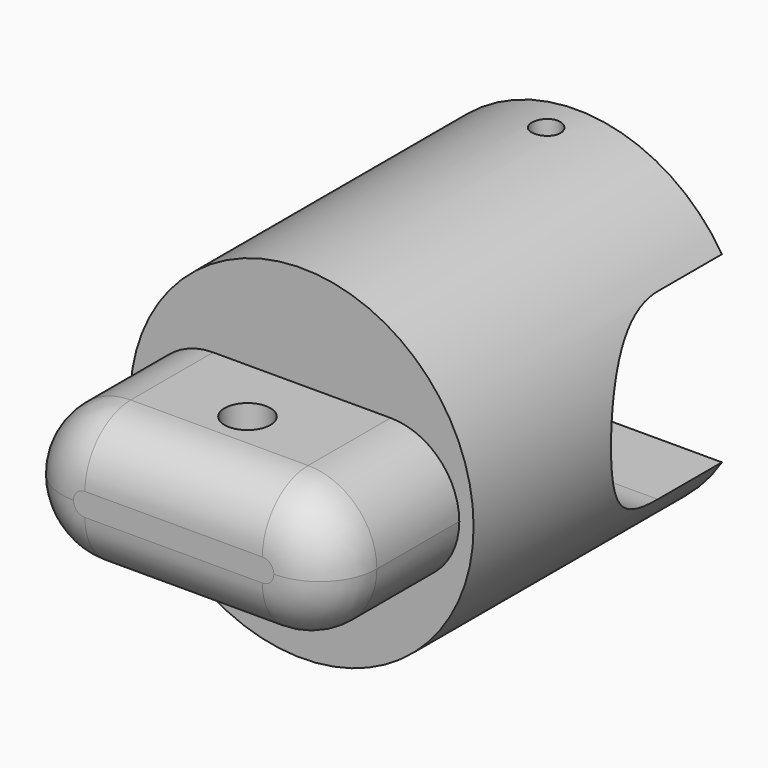
from build123d import *

# Parameters (mm, degrees)
F0_R           = 15
F1_DEPTH       = 30
F3_DEPTH       = 25
F3_DEPTH_BACK  = 25
F5_DEPTH       = 14
F6_R           = 5
F7_R           = 2
F8_DEPTH       = 25
F8_DEPTH_BACK  = 25
F9_R           = 1.25
F10_DEPTH      = 25
F10_DEPTH_BACK = 25


with BuildPart() as f1:
    # F0 (on Front) → F1 (new body)
    with BuildSketch(Plane.XZ):
        Circle(F0_R)
    extrude(amount=F1_DEPTH)

    # F2 (on Right) → F3 (cut, two sides)
    with BuildSketch(Plane.YZ) as f3_sk:
        with BuildLine():
            Line((15, 8), (-7, 8))
            ThreePointArc((-7, 8), (-12.6568542495, 5.6568542495), (-15, 0))
            ThreePointArc((-15, 0), (-12.6568542495, -5.6568542495), (-7, -8))
            Line((-7, -8), (15, -8))
            Line((15, -8), (15, 8))
        make_face()
    extrude(amount=-F3_DEPTH, mode=Mode.SUBTRACT)
    extrude(f3_sk.sketch, amount=F3_DEPTH_BACK, mode=Mode.SUBTRACT)

    # F4 (on face) → F5 (join)
    with BuildSketch(Plane.XZ.offset(30)):
        with BuildLine():
            ThreePointArc((13.7477270849, 0), (11.990367772, 4.2426406871), (7.7477270849, 6))
            Line((7.7477270849, 6), (-7.7477270849, 6))
            ThreePointArc((-7.7477270849, 6), (-11.990367772, 4.2426406871), (-13.7477270849, 0))
            ThreePointArc((-13.7477270849, 0), (-11.990367772, -4.2426406871), (-7.7477270849, -6))
            Line((-7.7477270849, -6), (7.7477270849, -6))
            ThreePointArc((7.7477270849, -6), (11.990367772, -4.2426406871), (13.7477270849, 0))
        make_face()
    extrude(amount=F5_DEPTH)

    # F6
    f6_edges = [f1.edges().sort_by_distance(p)[0] for p in [
        (13.747727, -44, 0),
        (0, -44, 6),
        (-13.747727, -44, 0),
        (0, -44, -6),
    ]]
    fillet(f6_edges, radius=F6_R)

    # F7 (on Top) → F8 (cut, two sides)
    with BuildSketch(Plane.XY) as f8_sk:
        with Locations((0, -35.9389074147)):
            Circle(F7_R)
    extrude(amount=-F8_DEPTH, mode=Mode.SUBTRACT)
    extrude(f8_sk.sketch, amount=F8_DEPTH_BACK, mode=Mode.SUBTRACT)

    # F9 (on Top) → F10 (cut, two sides)
    with BuildSketch(Plane.XY) as f10_sk:
        with Locations((0, -3.3346442506)):
            Circle(F9_R)
    extrude(amount=-F10_DEPTH, mode=Mode.SUBTRACT)
    extrude(f10_sk.sketch, amount=F10_DEPTH_BACK, mode=Mode.SUBTRACT)


solid = f1.part
